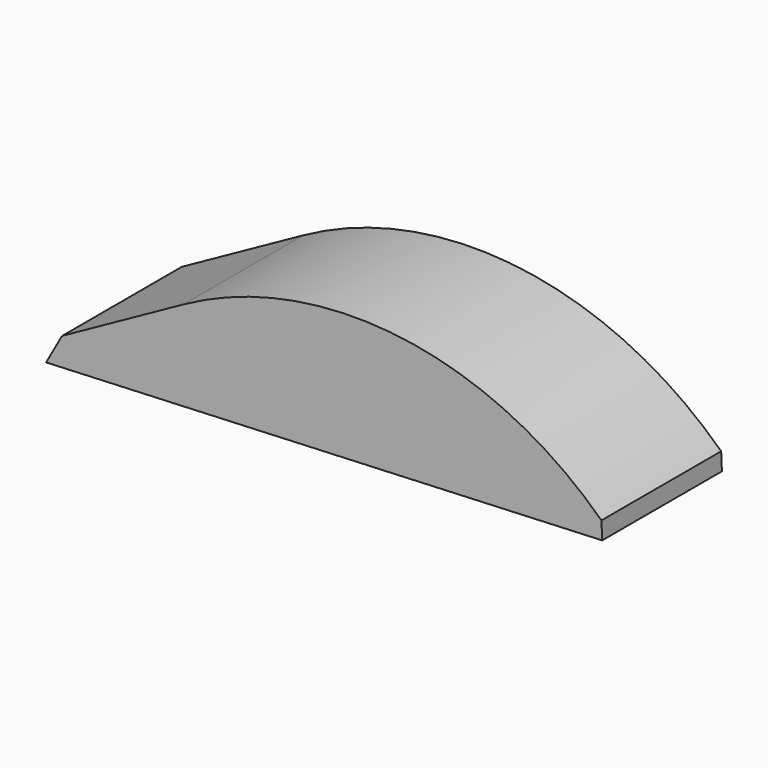
from build123d import *

# Parameters (mm, degrees)
F1_DEPTH    = 32.766
F2_T1_DEPTH = 555.7105242514
F3_DEPTH    = 3.81
F4_T1_DEPTH = 59.0353369856


# Not quite as in the source:
# - a fillet or chamfer that OpenCascade refuses, or shapes differently, is made with other operations: its cross-section is extruded or revolved along the edge and cut away or added


with BuildPart() as f1:
    # F0 (on Front) → F1 (new body)
    with BuildSketch(Plane.XZ):
        Polygon((57.8652285039, 0), (57.8652285039, 62.5251382589), (-64.6729022264, -5.3159417585), align=None)
    extrude(amount=F1_DEPTH)

    # F2: fillet of radius 77.8169467068 on 1 edges, made by hand

    # F2_s2 → F2_t1 (cut)
    with BuildSketch(Plane.XZ.offset(-261.4722621257)):
        with BuildLine():
            ThreePointArc((57.8652285039, 0), (14.0628423673, 20.9577145427), (-33.6365297354, 11.8667997855))
            Line((-33.6365297354, 11.8667997855), (-34.3903529504, 13.228394967))
            Line((-34.3903529504, 13.228394967), (57.111405289, 63.8867334405))
            Line((57.111405289, 63.8867334405), (59.4215674381, 62.5251382589))
            ThreePointArc((59.4215674381, 62.5251382589), (59.4215674381, 31.2625691295), (58.9414404538, 1.1242591859))
            Line((58.9414404538, 1.1242591859), (57.8652285039, 0))
        make_face()
    extrude(amount=F2_T1_DEPTH, mode=Mode.SUBTRACT)

    # F3 (add): a face of the model
    f3_faces = [f1.faces().sort_by_distance(p)[0] for p in [
        (-3.4038368613, -16.383, -2.6579708792),
    ]]
    extrude(f3_faces, amount=F3_DEPTH)

    # F4: chamfer of 5.08 on 1 edges, made by hand

    # F4_s2 → F4_t1 (cut)
    with BuildSketch(Plane.XZ.offset(-13.1346684928)):
        Polygon((-60.2285595639, -2.8554096417), (-64.4527290592, -10.3911682338), (-64.6729022264, -5.3159417585), align=None)
    extrude(amount=F4_T1_DEPTH, mode=Mode.SUBTRACT)


solid = f1.part
